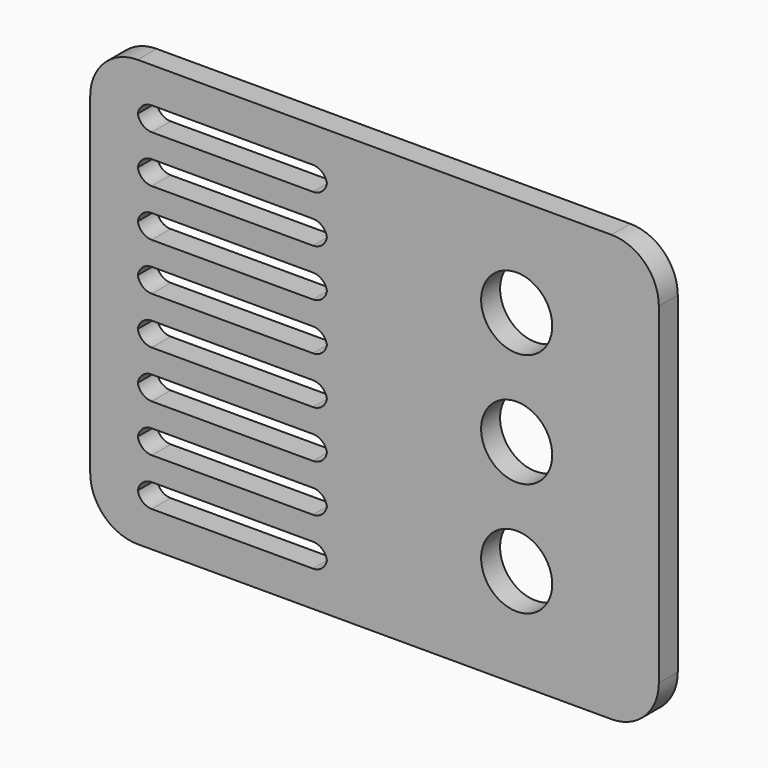
from build123d import *

# Parameters (mm, degrees)
F0_W         = 152.4
F0_H         = 114.3
F1_DEPTH     = 6.35
F2_R         = 12.7
F3_R         = 9.525
F4_DEPTH     = 25.4
F5_R         = 9.525
F6_DEPTH     = 25.4
F7_R         = 9.525
F8_DEPTH     = 25.4
F16_W        = 50.8
F16_H        = 6.35
F15_W        = 50.8
F15_H        = 6.35
F14_W        = 50.8
F14_H        = 6.35
F13_W        = 50.8
F13_H        = 6.35
F12_W        = 50.8
F12_H        = 6.35
F11_W        = 50.8
F11_H        = 6.35
F10_W        = 50.8
F10_H        = 6.35
F9_W         = 50.8
F9_H         = 6.35
F17_DEPTH    = 25.4
F18_T1_DEPTH = 6.35
F19_T1_DEPTH = 6.35


# Not quite as in the source:
# - a fillet or chamfer that OpenCascade refuses, or shapes differently, is made with other operations: its cross-section is extruded or revolved along the edge and cut away or added


with BuildPart() as f1:
    # F0 (on Front) → F1 (new body)
    with BuildSketch(Plane.XZ):
        Rectangle(F0_W, F0_H)
    extrude(amount=F1_DEPTH)

    # F2
    f2_edges = [f1.edges().sort_by_distance(p)[0] for p in [
        (-76.2, -3.175, 57.15),
        (-76.2, -3.175, -57.15),
        (76.2, -3.175, -57.15),
        (76.2, -3.175, 57.15),
    ]]
    fillet(f2_edges, radius=F2_R)

    # F3 (on face) → F4 (cut)
    with BuildSketch(Plane.XZ.offset(6.35)):
        with Locations((38.1, 30.48)):
            Circle(F3_R)
    extrude(amount=-F4_DEPTH, mode=Mode.SUBTRACT)

    # F5 (on face) → F6 (cut)
    with BuildSketch(Plane.XZ.offset(6.35)):
        with Locations((38.1, 0)):
            Circle(F5_R)
    extrude(amount=-F6_DEPTH, mode=Mode.SUBTRACT)

    # F7 (on face) → F8 (cut)
    with BuildSketch(Plane.XZ.offset(6.35)):
        with Locations((38.1, -30.48)):
            Circle(F7_R)
    extrude(amount=-F8_DEPTH, mode=Mode.SUBTRACT)

    # F16 (on face) + F15 (on face) + F14 (on face) + F13 (on face) + F12 (on face) + F11 (on face) + F10 (on face) + F9 (on face) → F17 (cut)
    with BuildSketch(Plane.XZ.offset(6.35)):
        with Locations((-38.1, 44.45)):
            Rectangle(F16_W, F16_H)
    with BuildSketch(Plane.XZ.offset(6.35)):
        with Locations((-38.1, 31.75)):
            Rectangle(F15_W, F15_H)
    with BuildSketch(Plane.XZ.offset(6.35)):
        with Locations((-38.1, 19.05)):
            Rectangle(F14_W, F14_H)
    with BuildSketch(Plane.XZ.offset(6.35)):
        with Locations((-38.1, 6.35)):
            Rectangle(F13_W, F13_H)
    with BuildSketch(Plane.XZ.offset(6.35)):
        with Locations((-38.1, -6.35)):
            Rectangle(F12_W, F12_H)
    with BuildSketch(Plane.XZ.offset(6.35)):
        with Locations((-38.1, -19.05)):
            Rectangle(F11_W, F11_H)
    with BuildSketch(Plane.XZ.offset(6.35)):
        with Locations((-38.1, -31.75)):
            Rectangle(F10_W, F10_H)
    with BuildSketch(Plane.XZ.offset(6.35)):
        with Locations((-38.1, -44.45)):
            Rectangle(F9_W, F9_H)
    extrude(amount=-F17_DEPTH, mode=Mode.SUBTRACT)

    # F18: fillet of radius 3.81 on 16 edges, made by hand

    # F18_s2 → F18_t1 (join)
    with BuildSketch(Plane.XZ):
        with BuildLine():
            ThreePointArc((-12.7, 6.985), (-13.8159231637, 4.2909231637), (-16.51, 3.175))
            Line((-16.51, 3.175), (-12.7, 3.175))
            Line((-12.7, 3.175), (-12.7, 6.985))
        make_face()
        with BuildLine():
            ThreePointArc((-16.51, -9.525), (-13.8159231637, -8.4090768363), (-12.7, -5.715))
            Line((-12.7, -5.715), (-12.7, -9.525))
            Line((-12.7, -9.525), (-16.51, -9.525))
        make_face()
        with BuildLine():
            ThreePointArc((-12.7, -31.115), (-13.8159231637, -33.8090768363), (-16.51, -34.925))
            Line((-16.51, -34.925), (-12.7, -34.925))
            Line((-12.7, -34.925), (-12.7, -31.115))
        make_face()
        with BuildLine():
            ThreePointArc((-16.51, -22.225), (-13.8159231637, -21.1090768363), (-12.7, -18.415))
            Line((-12.7, -18.415), (-12.7, -22.225))
            Line((-12.7, -22.225), (-16.51, -22.225))
        make_face()
        with BuildLine():
            ThreePointArc((-12.7, -43.815), (-13.8159231637, -46.5090768363), (-16.51, -47.625))
            Line((-16.51, -47.625), (-12.7, -47.625))
            Line((-12.7, -47.625), (-12.7, -43.815))
        make_face()
        with BuildLine():
            ThreePointArc((-16.51, 15.875), (-13.8159231637, 16.9909231637), (-12.7, 19.685))
            Line((-12.7, 19.685), (-12.7, 15.875))
            Line((-12.7, 15.875), (-16.51, 15.875))
        make_face()
        with BuildLine():
            ThreePointArc((-16.51, 28.575), (-13.8159231637, 29.6909231637), (-12.7, 32.385))
            Line((-12.7, 32.385), (-12.7, 28.575))
            Line((-12.7, 28.575), (-16.51, 28.575))
        make_face()
        with BuildLine():
            ThreePointArc((-16.51, 41.275), (-13.8159231637, 42.3909231637), (-12.7, 45.085))
            Line((-12.7, 45.085), (-12.7, 41.275))
            Line((-12.7, 41.275), (-16.51, 41.275))
        make_face()
        with BuildLine():
            ThreePointArc((-12.7, -45.085), (-13.8159231637, -42.3909231637), (-16.51, -41.275))
            Line((-16.51, -41.275), (-12.7, -41.275))
            Line((-12.7, -41.275), (-12.7, -45.085))
        make_face()
        with BuildLine():
            ThreePointArc((-12.7, -32.385), (-13.8159231637, -29.6909231637), (-16.51, -28.575))
            Line((-16.51, -28.575), (-12.7, -28.575))
            Line((-12.7, -28.575), (-12.7, -32.385))
        make_face()
        with BuildLine():
            ThreePointArc((-12.7, -19.685), (-13.8159231637, -16.9909231637), (-16.51, -15.875))
            Line((-16.51, -15.875), (-12.7, -15.875))
            Line((-12.7, -15.875), (-12.7, -19.685))
        make_face()
        with BuildLine():
            ThreePointArc((-12.7, -6.985), (-13.8159231637, -4.2909231637), (-16.51, -3.175))
            Line((-16.51, -3.175), (-12.7, -3.175))
            Line((-12.7, -3.175), (-12.7, -6.985))
        make_face()
        with BuildLine():
            ThreePointArc((-12.7, 5.715), (-13.8159231637, 8.4090768363), (-16.51, 9.525))
            Line((-16.51, 9.525), (-12.7, 9.525))
            Line((-12.7, 9.525), (-12.7, 5.715))
        make_face()
        with BuildLine():
            ThreePointArc((-12.7, 18.415), (-13.8159231637, 21.1090768363), (-16.51, 22.225))
            Line((-16.51, 22.225), (-12.7, 22.225))
            Line((-12.7, 22.225), (-12.7, 18.415))
        make_face()
        with BuildLine():
            ThreePointArc((-12.7, 31.115), (-13.8159231637, 33.8090768363), (-16.51, 34.925))
            Line((-16.51, 34.925), (-12.7, 34.925))
            Line((-12.7, 34.925), (-12.7, 31.115))
        make_face()
        with BuildLine():
            ThreePointArc((-12.7, 43.815), (-13.8159231637, 46.5090768363), (-16.51, 47.625))
            Line((-16.51, 47.625), (-12.7, 47.625))
            Line((-12.7, 47.625), (-12.7, 43.815))
        make_face()
    extrude(amount=F18_T1_DEPTH)

    # F19: fillet of radius 3.81 on 16 edges, made by hand

    # F19_s2 → F19_t1 (join)
    with BuildSketch(Plane.XZ):
        with BuildLine():
            ThreePointArc((-59.69, 47.625), (-62.3840768363, 46.5090768363), (-63.5, 43.815))
            Line((-63.5, 43.815), (-63.5, 47.625))
            Line((-63.5, 47.625), (-59.69, 47.625))
        make_face()
        with BuildLine():
            ThreePointArc((-59.69, 34.925), (-62.3840768363, 33.8090768363), (-63.5, 31.115))
            Line((-63.5, 31.115), (-63.5, 34.925))
            Line((-63.5, 34.925), (-59.69, 34.925))
        make_face()
        with BuildLine():
            ThreePointArc((-59.69, 22.225), (-62.3840768363, 21.1090768363), (-63.5, 18.415))
            Line((-63.5, 18.415), (-63.5, 22.225))
            Line((-63.5, 22.225), (-59.69, 22.225))
        make_face()
        with BuildLine():
            ThreePointArc((-59.69, 9.525), (-62.3840768363, 8.4090768363), (-63.5, 5.715))
            Line((-63.5, 5.715), (-63.5, 9.525))
            Line((-63.5, 9.525), (-59.69, 9.525))
        make_face()
        with BuildLine():
            ThreePointArc((-59.69, -3.175), (-62.3840768363, -4.2909231637), (-63.5, -6.985))
            Line((-63.5, -6.985), (-63.5, -3.175))
            Line((-63.5, -3.175), (-59.69, -3.175))
        make_face()
        with BuildLine():
            ThreePointArc((-59.69, -15.875), (-62.3840768363, -16.9909231637), (-63.5, -19.685))
            Line((-63.5, -19.685), (-63.5, -15.875))
            Line((-63.5, -15.875), (-59.69, -15.875))
        make_face()
        with BuildLine():
            ThreePointArc((-59.69, -28.575), (-62.3840768363, -29.6909231637), (-63.5, -32.385))
            Line((-63.5, -32.385), (-63.5, -28.575))
            Line((-63.5, -28.575), (-59.69, -28.575))
        make_face()
        with BuildLine():
            ThreePointArc((-59.69, -41.275), (-62.3840768363, -42.3909231637), (-63.5, -45.085))
            Line((-63.5, -45.085), (-63.5, -41.275))
            Line((-63.5, -41.275), (-59.69, -41.275))
        make_face()
        with BuildLine():
            ThreePointArc((-59.69, 41.275), (-62.3840768363, 42.3909231637), (-63.5, 45.085))
            Line((-63.5, 45.085), (-63.5, 41.275))
            Line((-63.5, 41.275), (-59.69, 41.275))
        make_face()
        with BuildLine():
            ThreePointArc((-59.69, 28.575), (-62.3840768363, 29.6909231637), (-63.5, 32.385))
            Line((-63.5, 32.385), (-63.5, 28.575))
            Line((-63.5, 28.575), (-59.69, 28.575))
        make_face()
        with BuildLine():
            ThreePointArc((-59.69, 15.875), (-62.3840768363, 16.9909231637), (-63.5, 19.685))
            Line((-63.5, 19.685), (-63.5, 15.875))
            Line((-63.5, 15.875), (-59.69, 15.875))
        make_face()
        with BuildLine():
            ThreePointArc((-63.5, 6.985), (-62.3840768363, 4.2909231637), (-59.69, 3.175))
            Line((-59.69, 3.175), (-63.5, 3.175))
            Line((-63.5, 3.175), (-63.5, 6.985))
        make_face()
        with BuildLine():
            ThreePointArc((-59.69, -9.525), (-62.3840768363, -8.4090768363), (-63.5, -5.715))
            Line((-63.5, -5.715), (-63.5, -9.525))
            Line((-63.5, -9.525), (-59.69, -9.525))
        make_face()
        with BuildLine():
            ThreePointArc((-59.69, -22.225), (-62.3840768363, -21.1090768363), (-63.5, -18.415))
            Line((-63.5, -18.415), (-63.5, -22.225))
            Line((-63.5, -22.225), (-59.69, -22.225))
        make_face()
        with BuildLine():
            ThreePointArc((-63.5, -31.115), (-62.3840768363, -33.8090768363), (-59.69, -34.925))
            Line((-59.69, -34.925), (-63.5, -34.925))
            Line((-63.5, -34.925), (-63.5, -31.115))
        make_face()
        with BuildLine():
            ThreePointArc((-63.5, -43.815), (-62.3840768363, -46.5090768363), (-59.69, -47.625))
            Line((-59.69, -47.625), (-63.5, -47.625))
            Line((-63.5, -47.625), (-63.5, -43.815))
        make_face()
    extrude(amount=F19_T1_DEPTH)


solid = f1.part
